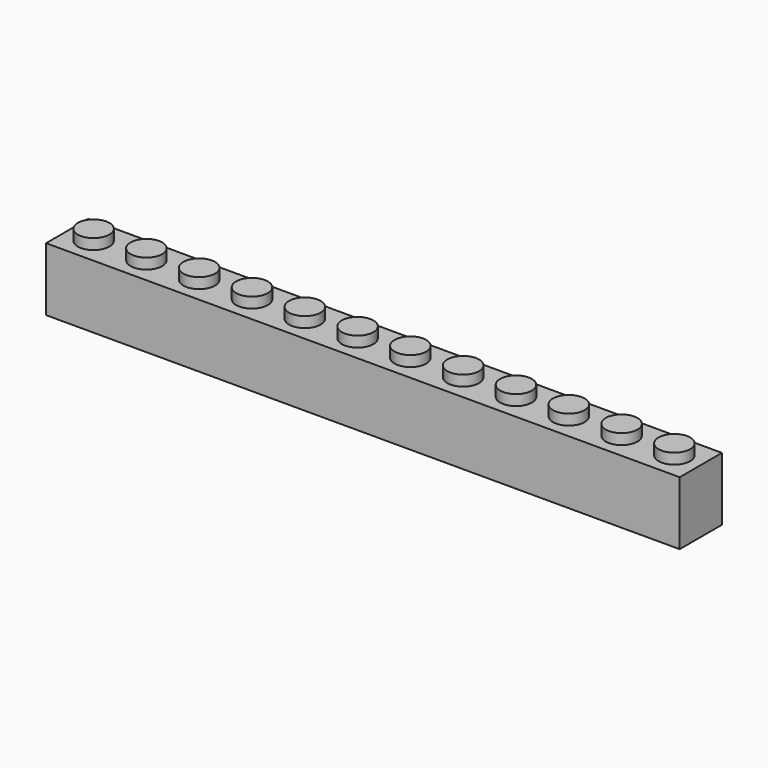
from build123d import *

# Parameters (mm, degrees)
F0_W     = 95.25
F0_H     = 7.9375
F0_R     = 2.38125
F1_DEPTH = 9.525
F2_DEPTH = 11.1125
F3_T     = -1.5875
F4_R     = 1.5875
F4_R_2   = 0.79375
F5_DEPTH = 7.9375


# Not quite as in the source:
# - a feature names something its author has since deleted; it is built from what else it names


with BuildPart() as f1:
    # F0 (on Top) → F1 (new body)
    with BuildSketch(Plane.XY):
        Rectangle(F0_W, F0_H)
        with Locations((-43.65625, 0)):
            Circle(F0_R, mode=Mode.SUBTRACT)
        with Locations((-35.71875, 0)):
            Circle(F0_R, mode=Mode.SUBTRACT)
        with Locations((-27.78125, 0)):
            Circle(F0_R, mode=Mode.SUBTRACT)
        with Locations((-19.84375, 0)):
            Circle(F0_R, mode=Mode.SUBTRACT)
        with Locations((-11.90625, 0)):
            Circle(F0_R, mode=Mode.SUBTRACT)
        with Locations((-3.96875, 0)):
            Circle(F0_R, mode=Mode.SUBTRACT)
        with Locations((3.96875, 0)):
            Circle(F0_R, mode=Mode.SUBTRACT)
        with Locations((11.90625, 0)):
            Circle(F0_R, mode=Mode.SUBTRACT)
        with Locations((19.84375, 0)):
            Circle(F0_R, mode=Mode.SUBTRACT)
        with Locations((27.78125, 0)):
            Circle(F0_R, mode=Mode.SUBTRACT)
        with Locations((35.71875, 0)):
            Circle(F0_R, mode=Mode.SUBTRACT)
        with Locations((43.65625, 0)):
            Circle(F0_R, mode=Mode.SUBTRACT)
    extrude(amount=F1_DEPTH)

    # F0 (on Top) → F2 (join)
    with BuildSketch(Plane.XY):
        with Locations((-43.65625, 0)):
            Circle(F0_R)
        with Locations((-35.71875, 0)):
            Circle(F0_R)
        with Locations((-27.78125, 0)):
            Circle(F0_R)
        with Locations((-19.84375, 0)):
            Circle(F0_R)
        with Locations((-11.90625, 0)):
            Circle(F0_R)
        with Locations((-3.96875, 0)):
            Circle(F0_R)
        with Locations((3.96875, 0)):
            Circle(F0_R)
        with Locations((11.90625, 0)):
            Circle(F0_R)
        with Locations((19.84375, 0)):
            Circle(F0_R)
        with Locations((27.78125, 0)):
            Circle(F0_R)
        with Locations((35.71875, 0)):
            Circle(F0_R)
        with Locations((43.65625, 0)):
            Circle(F0_R)
    extrude(amount=F2_DEPTH)

    # F3
    f3_openings = [f1.faces().sort_by_distance(p)[0] for p in [
        (0, 0, 0),
    ]]
    offset(amount=F3_T, openings=f3_openings, kind=Kind.INTERSECTION)

    # F4 (on face) → F5 (join)
    with BuildSketch(Plane(origin=(0, 0, 7.9375), x_dir=(1, 0, 0), z_dir=(0, 0, -1))):
        with Locations((-39.6875, 0)):
            Circle(F4_R)
        with Locations((-39.6875, 0)):
            Circle(F4_R_2, mode=Mode.SUBTRACT)
        with Locations((-31.75, 0)):
            Circle(F4_R)
        with Locations((-31.75, 0)):
            Circle(F4_R_2, mode=Mode.SUBTRACT)
        with Locations((-23.8125, 0)):
            Circle(F4_R)
        with Locations((-23.8125, 0)):
            Circle(F4_R_2, mode=Mode.SUBTRACT)
        with Locations((-15.875, 0)):
            Circle(F4_R)
        with Locations((-15.875, 0)):
            Circle(F4_R_2, mode=Mode.SUBTRACT)
        with Locations((-7.9375, 0)):
            Circle(F4_R)
        with Locations((-7.9375, 0)):
            Circle(F4_R_2, mode=Mode.SUBTRACT)
        Circle(F4_R)
        Circle(F4_R_2, mode=Mode.SUBTRACT)
        with Locations((7.9375, 0)):
            Circle(F4_R)
        with Locations((7.9375, 0)):
            Circle(F4_R_2, mode=Mode.SUBTRACT)
        with Locations((15.875, 0)):
            Circle(F4_R)
        with Locations((15.875, 0)):
            Circle(F4_R_2, mode=Mode.SUBTRACT)
        with Locations((23.8125, 0)):
            Circle(F4_R)
        with Locations((23.8125, 0)):
            Circle(F4_R_2, mode=Mode.SUBTRACT)
        with Locations((31.75, 0)):
            Circle(F4_R)
        with Locations((31.75, 0)):
            Circle(F4_R_2, mode=Mode.SUBTRACT)
        with Locations((39.6875, 0)):
            Circle(F4_R)
        with Locations((39.6875, 0)):
            Circle(F4_R_2, mode=Mode.SUBTRACT)
    extrude(amount=F5_DEPTH)


solid = f1.part
